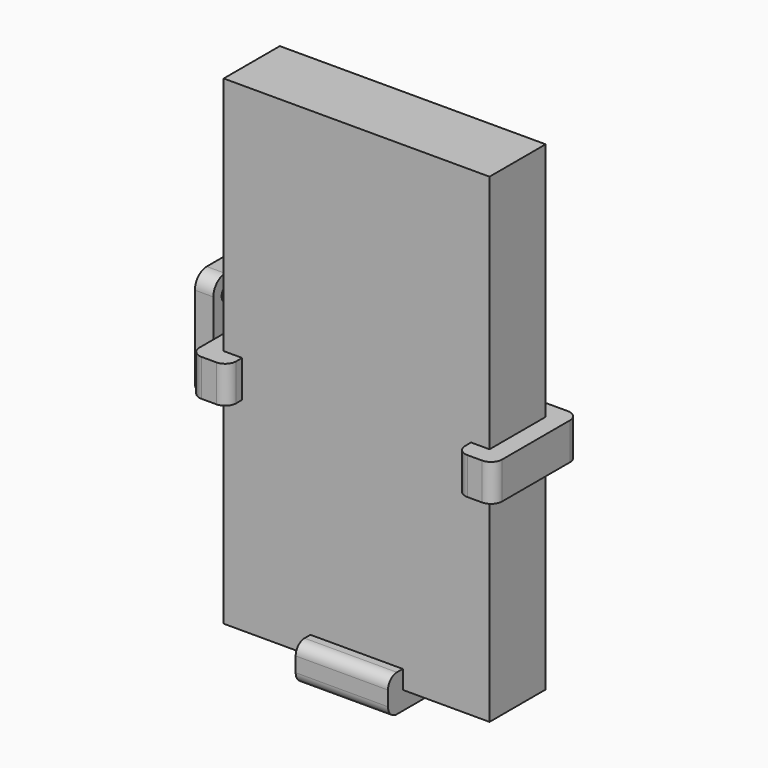
from build123d import *

# Parameters (mm, degrees)
F0_W      = 72
F0_H      = 130
F1_DEPTH  = 19
F3_DEPTH  = 12.5
F4_R      = 3
F6_DEPTH  = 10
F7_R      = 3
F8_W      = 10
F8_H      = 5
F9_DEPTH  = 10
F10_R     = 2.2
F11_DEPTH = 5
F12_R     = 4
F14_START = 10
F14_DEPTH = 15


# Not quite as in the source:
# - a pattern or mirror of a feature is missing from the dataset's text; its kind, count and spacing are read off the source's solid


with BuildPart() as f1:
    # F0 (on Front) → F1 (new body)
    with BuildSketch(Plane.XZ):
        Rectangle(F0_W, F0_H)
    extrude(amount=F1_DEPTH)


with BuildPart() as f3:
    # F2 (on Right) → F3 (new body, symmetric)
    with BuildSketch(Plane.YZ):
        Polygon((5, 0), (0, 0), (0, -65), (-19, -65), (-19, -60), (-24, -60), (-24, -70), (5, -70), align=None)
    extrude(amount=F3_DEPTH, both=True)

    # F4
    f4_edges = [f3.edges().sort_by_distance(p)[0] for p in [
        (0, -24, -60),
        (0, -24, -70),
        (0, 5, -70),
    ]]
    fillet(f4_edges, radius=F4_R)

    # F5 (on Top) → F6 (join)
    with BuildSketch(Plane.XY):
        Polygon((12.5, 5), (12.5, 0), (36, 0), (36, -19), (31, -19), (31, -24), (41, -24), (41, 5), align=None)
        Polygon((-12.5, 0), (-12.5, 5), (-41, 5), (-41, -24), (-31, -24), (-31, -19), (-36, -19), (-36, 0), align=None)
    extrude(amount=-F6_DEPTH)

    # F7
    f7_edges = [f3.edges().sort_by_distance(p)[0] for p in [
        (31, -24, -5),
        (41, -24, -5),
        (41, 5, -5),
        (-41, -24, -5),
        (-31, -24, -5),
    ]]
    fillet(f7_edges, radius=F7_R)

    # F8 (on Top) → F9 (join, through all)
    with BuildSketch(Plane.XY):
        with Locations((-46, 2.5)):
            Rectangle(F8_W, F8_H)
    extrude(amount=-F9_DEPTH)

    # F10 (on face) → F11 (join)
    with BuildSketch(Plane(origin=(-51, 0, 0), x_dir=(0, -1, 0), z_dir=(-1, 0, 0))):
        Polygon((10, 10), (-5, 10), (-5, 0), (0, 0), (0, -10), (-5, -10), (-5, -20), (10, -20), align=None)
        with Locations((5, -15)):
            Circle(F10_R, mode=Mode.SUBTRACT)
        with Locations((5, 5)):
            Circle(F10_R, mode=Mode.SUBTRACT)
    extrude(amount=-F11_DEPTH)

    # F12
    f12_edges = [f3.edges().sort_by_distance(p)[0] for p in [
        (-48.5, -10, 10),
        (-48.5, -10, -20),
        (-48.5, 5, 10),
        (-48.5, 5, -20),
    ]]
    fillet(f12_edges, radius=F12_R)

    # F13 (on Right) → F14 (join)
    with BuildSketch(Plane.YZ.offset(F14_START)):
        with BuildLine():
            Line((0, 4.1183650965), (0, 0))
            Line((0, 0), (5, 0))
            Line((5, 0), (5, 13.2424322584))
            Line((5, 13.2424322584), (3, 13.2424322584))
            Line((3, 13.2424322584), (0.3015368961, 5.8284658131))
            ThreePointArc((0.3015368961, 5.8284658131), (0.0759612349, 4.9866059848), (0, 4.1183650965))
        make_face()
    f14 = extrude(amount=F14_DEPTH)

    # F14_copies: F14 across plane
    add(f14.mirror(Plane(origin=(0, 0, 0), x_dir=(0, 0, -1), z_dir=(-1, 0, 0))))


solid = Compound([f1.part, f3.part])
